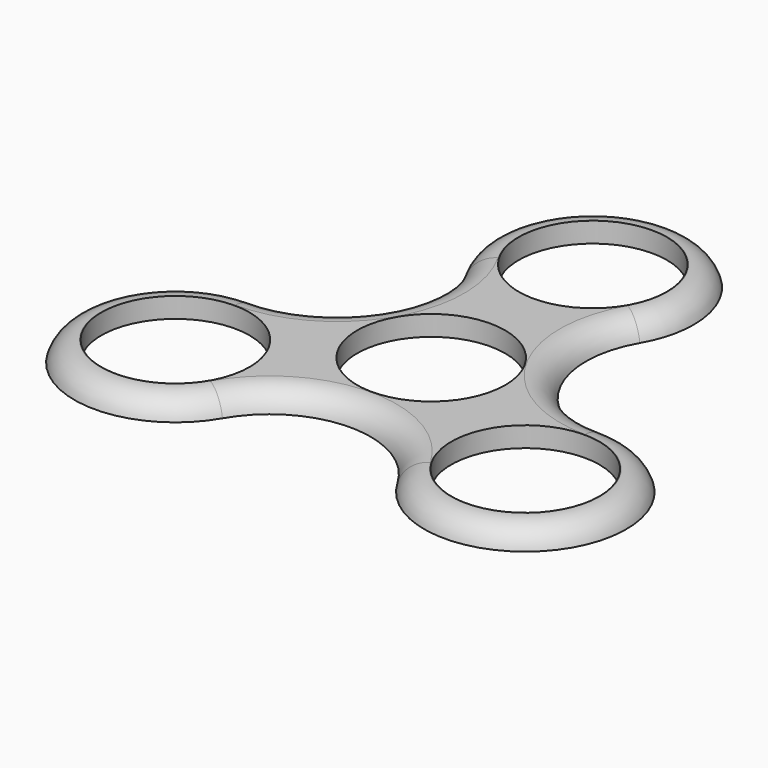
from build123d import *

# Parameters (mm, degrees)
F0_R         = 11
F1_DEPTH     = 3
F2_T2_ANGLE  = 120
F2_T4_ANGLE  = 240
F2_T6_ANGLE  = 240
F2_T8_ANGLE  = 120
F2_T10_ANGLE = 240
F2_T12_ANGLE = 120


# Not quite as in the source:
# - a fillet or chamfer that OpenCascade refuses, or shapes differently, is made with other operations: its cross-section is extruded or revolved along the edge and cut away or added


with BuildPart() as f1:
    # F0 (on Top) → F1 (new body)
    with BuildSketch(Plane.XY):
        with BuildLine():
            ThreePointArc((12.9903810568, 22.5), (14.4888873943, 26.1177143235), (15, 30))
            ThreePointArc((15, 30), (-3.8822856765, 44.4888873943), (-12.9903810568, 22.5))
            ThreePointArc((-12.9903810568, 22.5), (0, 15), (12.9903810568, 22.5))
        make_face()
        with Locations((0, 30)):
            Circle(F0_R, mode=Mode.SUBTRACT)
        with BuildLine():
            ThreePointArc((12.9903810568, 22.5), (0, 15), (-12.9903810568, 22.5))
            ThreePointArc((-12.9903810568, 22.5), (-12.9903810568, 7.5), (-25.9807621135, 0))
            ThreePointArc((-25.9807621135, 0), (-15.3741603957, -4.3933982822), (-10.9807621135, -15))
            ThreePointArc((-10.9807621135, -15), (-11.4918747192, -18.8822856765), (-12.9903810568, -22.5))
            ThreePointArc((-12.9903810568, -22.5), (0, -15), (12.9903810568, -22.5))
            ThreePointArc((12.9903810568, -22.5), (12.9903810568, -7.5), (25.9807621135, 0))
            ThreePointArc((25.9807621135, 0), (12.9903810568, 7.5), (12.9903810568, 22.5))
        make_face()
        Circle(F0_R, mode=Mode.SUBTRACT)
        with BuildLine():
            ThreePointArc((-10.9807621135, -15), (-15.3741603957, -4.3933982822), (-25.9807621135, 0))
            ThreePointArc((-25.9807621135, 0), (-38.9711431703, -22.5), (-12.9903810568, -22.5))
            ThreePointArc((-12.9903810568, -22.5), (-11.4918747192, -18.8822856765), (-10.9807621135, -15))
        make_face()
        with Locations((-25.9807621135, -15)):
            Circle(F0_R, mode=Mode.SUBTRACT)
        with BuildLine():
            ThreePointArc((40.9807621135, -15), (36.5873638313, -4.3933982822), (25.9807621135, 0))
            ThreePointArc((25.9807621135, 0), (12.9903810568, -7.5), (12.9903810568, -22.5))
            ThreePointArc((12.9903810568, -22.5), (29.8630477901, -29.4888873943), (40.9807621135, -15))
        make_face()
        with Locations((25.9807621135, -15)):
            Circle(F0_R, mode=Mode.SUBTRACT)
    extrude(amount=F1_DEPTH)

    # F2: fillet of radius 4 on 1 edges, made by hand

    # F2_s1 → F2_t2 (revolve, cut)
    with BuildSketch(Plane(origin=(-12.9903810568, 22.5, 0), x_dir=(0, 0, 1), z_dir=(-0.5, 0.8660254038, 0))):
        with BuildLine():
            ThreePointArc((0, 0), (2.1622776602, 1.4234936034), (3, 3.8729833462))
            Line((3, 3.8729833462), (3, 0))
            Line((3, 0), (0, 0))
        make_face()
    revolve(axis=Axis((-25.9807621135, 15, 3), (0, 0, -1)), revolution_arc=F2_T2_ANGLE, mode=Mode.SUBTRACT)

    # F2_s3 → F2_t4 (revolve, cut)
    with BuildSketch(Plane(origin=(12.9903810568, 22.5, 0), x_dir=(0, 0, 1), z_dir=(-0.5, -0.8660254038, 0))):
        with BuildLine():
            ThreePointArc((0, 0), (2.1622776602, 1.4234936034), (3, 3.8729833462))
            Line((3, 3.8729833462), (3, 0))
            Line((3, 0), (0, 0))
        make_face()
    revolve(axis=Axis((0, 30, 3), (0, 0, 1)), revolution_arc=F2_T4_ANGLE, mode=Mode.SUBTRACT)

    # F2_s5 → F2_t6 (revolve, cut)
    with BuildSketch(Plane.YZ.offset(-25.9807621135)):
        with BuildLine():
            ThreePointArc((0, 0), (-1.4234936034, 2.1622776602), (-3.8729833462, 3))
            Line((-3.8729833462, 3), (0, 3))
            Line((0, 3), (0, 0))
        make_face()
    revolve(axis=Axis((-25.9807621135, -15, 3), (0, 0, 1)), revolution_arc=F2_T6_ANGLE, mode=Mode.SUBTRACT)

    # F2_s7 → F2_t8 (revolve, cut)
    with BuildSketch(Plane(origin=(-12.9903810568, -22.5, 0), x_dir=(0, 0, 1), z_dir=(-0.5, -0.8660254038, 0))):
        with BuildLine():
            ThreePointArc((0, 0), (2.1622776602, 1.4234936034), (3, 3.8729833462))
            Line((3, 3.8729833462), (3, 0))
            Line((3, 0), (0, 0))
        make_face()
    revolve(axis=Axis((0, -30, 3), (0, 0, -1)), revolution_arc=F2_T8_ANGLE, mode=Mode.SUBTRACT)

    # F2_s9 → F2_t10 (revolve, cut)
    with BuildSketch(Plane(origin=(12.9903810568, -22.5, 0), x_dir=(0, 0, 1), z_dir=(-0.5, 0.8660254038, 0))):
        with BuildLine():
            ThreePointArc((0, 0), (2.1622776602, 1.4234936034), (3, 3.8729833462))
            Line((3, 3.8729833462), (3, 0))
            Line((3, 0), (0, 0))
        make_face()
    revolve(axis=Axis((25.9807621135, -15, 3), (0, 0, 1)), revolution_arc=F2_T10_ANGLE, mode=Mode.SUBTRACT)

    # F2_s11 → F2_t12 (revolve, cut)
    with BuildSketch(Plane.YZ.offset(25.9807621135)):
        with BuildLine():
            ThreePointArc((0, 0), (-1.4234936034, 2.1622776602), (-3.8729833462, 3))
            Line((-3.8729833462, 3), (0, 3))
            Line((0, 3), (0, 0))
        make_face()
    revolve(axis=Axis((25.9807621135, 15, 3), (0, 0, -1)), revolution_arc=F2_T12_ANGLE, mode=Mode.SUBTRACT)


solid = f1.part
